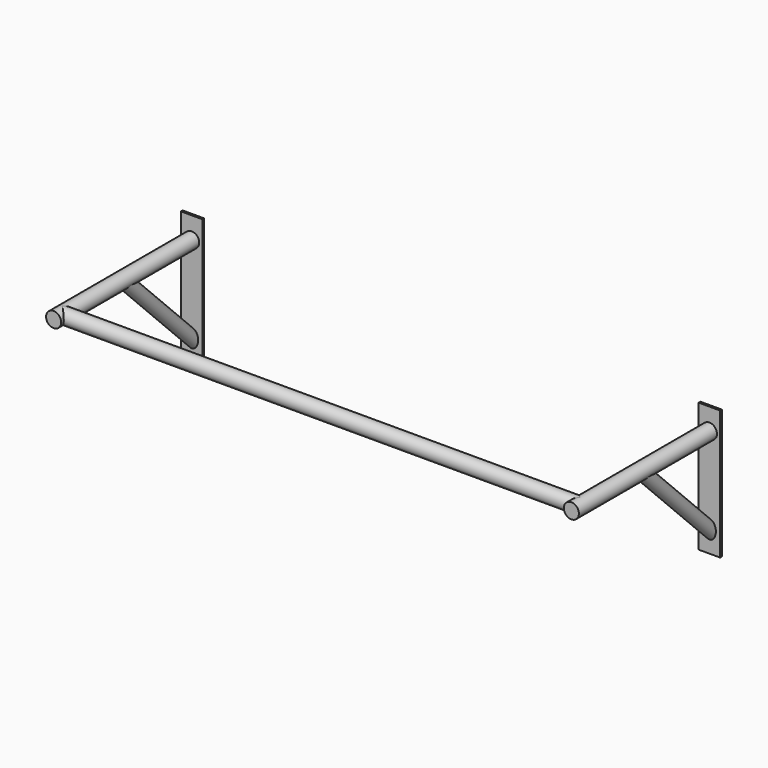
from build123d import *

# Parameters (mm, degrees)
F0_W      = 50
F0_H      = 300
F1_DEPTH  = 5
F2_R      = 17.5
F3_DEPTH  = 400
F7_R      = 15
F8_REACH  = 364.1609923111
F10_R     = 17.5
F11_DEPTH = 600


with BuildPart() as f1:
    # F0 (on Front) → F1 (new body)
    with BuildSketch(Plane.XZ):
        with Locations((-600, -100)):
            Rectangle(F0_W, F0_H)
    extrude(amount=F1_DEPTH)

    # F2 (on face) → F3 (join)
    with BuildSketch(Plane.XZ.offset(5)):
        with Locations((-600, 0)):
            Circle(F2_R)
    extrude(amount=F3_DEPTH)

    f8_end = f1.faces().sort_by_distance((-600, -5, -106.8536862637))[0]
    # F7 (on line) → F8 (join, up to a face of the model that its end follows)
    with BuildSketch(Plane(origin=(0, -102.5, 102.5), x_dir=(1, 0, 0), z_dir=(0, -0.7071067812, 0.7071067812))):
        with Locations((-600, -144.9568901432)):
            Circle(F7_R)
    f8_long = extrude(amount=-F8_REACH, mode=Mode.PRIVATE)
    add(split(f8_long, bisect_by=f8_end, keep=Keep.TOP, mode=Mode.PRIVATE))


with BuildPart() as f9_1:
    # F9: instance of F1
    add(f1.part.mirror(Plane.YZ))


with BuildPart() as f11:
    # F10 (on Right) → F11 (new body, symmetric)
    with BuildSketch(Plane.YZ):
        with Locations((-380, 0)):
            Circle(F10_R)
    extrude(amount=F11_DEPTH, both=True)


solid = Compound([f1.part, f9_1.part, f11.part])
